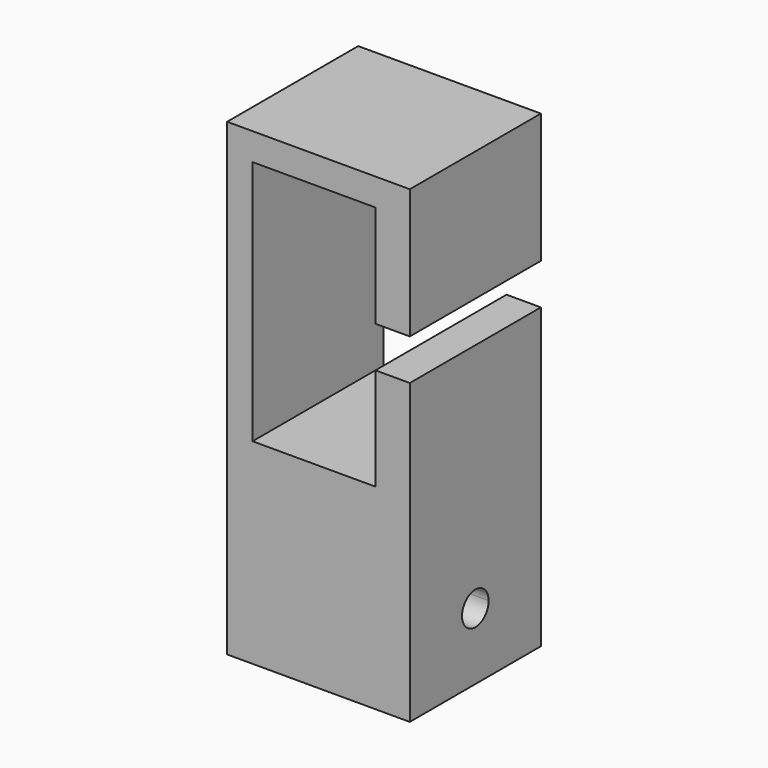
from build123d import *

# Parameters (mm, degrees)
F2_DEPTH = 25.4
F3_W     = 6.35
F3_H     = 25.4
F3_W_2   = 15.6204670995
F4_DEPTH = 25.4
F6_DEPTH = 38.1


# Not quite as in the source:
# - a feature names something its author has since deleted; it is built from what else it names


with BuildPart() as f2:
    # F1 (on offset) → F2 (new body)
    with BuildSketch(Plane.XZ.offset(25.4)):
        Polygon((-12.7, -19.4027777778), (-12.7, 18.6972222222), (6.35, 18.6972222222), (6.35, 2.8222222222), (11.6785410792, 2.8222222222), (11.6785410792, 22.9191370308), (-16.6419260204, 22.9191370308), (-16.6419260204, -24.3789628148), (11.6785410792, -24.3789628148), (11.6785410792, -3.5277777778), (6.35, -3.5277777778), (6.35, -19.4027777778), align=None)
    extrude(amount=F2_DEPTH)

    # F3 (on face) → F4 (join)
    with BuildSketch(Plane(origin=(0, 0, -24.3789628148), x_dir=(1, 0, 0), z_dir=(0, 0, -1))):
        with Locations((-13.4669260204, 38.1)):
            Rectangle(F3_W, F3_H)
        with Locations((8.5035410792, 38.1)):
            Rectangle(F3_W, F3_H)
        with Locations((-2.4816924706, 38.1)):
            Rectangle(F3_W_2, F3_H)
    extrude(amount=F4_DEPTH)

    # F5 (on face) → F6 (cut)
    with BuildSketch(Plane.YZ.offset(11.6785410792)):
        with BuildLine():
            ThreePointArc((-35.5203125, -39.4433777778), (-36.2758854754, -37.6192632532), (-38.1, -36.8636902778))
            ThreePointArc((-38.1, -36.8636902778), (-39.9241145246, -41.2674923024), (-35.5203125, -39.4433777778))
        make_face()
    extrude(amount=-F6_DEPTH, mode=Mode.SUBTRACT)


solid = f2.part
